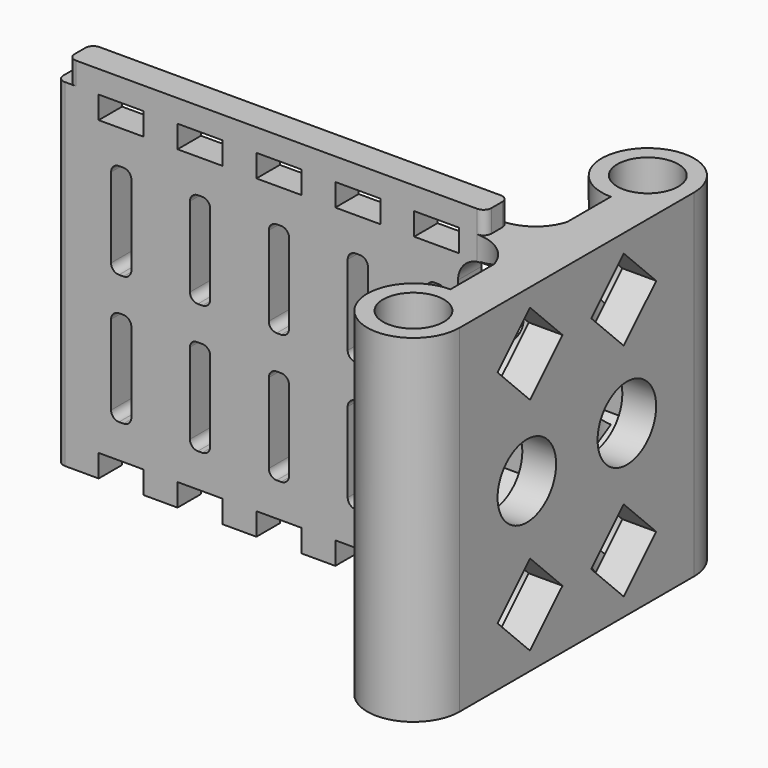
from build123d import *

# Parameters (mm, degrees)
F0_R     = 2.7
F1_DEPTH = 30
F3_DEPTH = 2
F4_R     = 3.25
F5_DEPTH = 25
F6_START = -3
F4_R_2   = 5
F6_DEPTH = 4.5
F7_W     = 4
F7_H     = 2
F8_DEPTH = 5


# Not quite as in the source:
# - a feature names something its author has since deleted; it is built from what else it names


with BuildPart() as f1:
    # F0 (on Top) → F1 (new body)
    with BuildSketch(Plane.XY):
        with BuildLine():
            ThreePointArc((14.1813559458, 17.5603501923), (17.0804937486, 18.7612123895), (18.2813559458, 21.6603501923))
            ThreePointArc((18.2813559458, 21.6603501923), (11.2822181429, 24.5594879952), (14.1813559458, 17.5603501923))
        make_face()
        with Locations((14.1813559458, 21.6603501923)):
            Circle(F0_R, mode=Mode.SUBTRACT)
        with BuildLine():
            Line((18.2813559458, -4.3396498077), (18.2813559458, 21.6603501923))
            ThreePointArc((18.2813559458, 21.6603501923), (17.0804937486, 18.7612123895), (14.1813559458, 17.5603501923))
            Line((14.1813559458, 17.5603501923), (14.1813559458, 12.7042196833))
            Line((14.1813559458, 12.7042196833), (14.1813559458, 4.6164807014))
            Line((14.1813559458, 4.6164807014), (14.1813559458, -0.2396498077))
            ThreePointArc((14.1813559458, -0.2396498077), (17.0804937486, -1.4405120048), (18.2813559458, -4.3396498077))
        make_face()
        with BuildLine():
            ThreePointArc((14.1813559458, -0.2396498077), (11.2822181429, -7.2387876105), (18.2813559458, -4.3396498077))
            ThreePointArc((18.2813559458, -4.3396498077), (17.0804937486, -1.4405120048), (14.1813559458, -0.2396498077))
        make_face()
        with Locations((14.1813559458, -4.3396498077)):
            Circle(F0_R, mode=Mode.SUBTRACT)
        with BuildLine():
            Line((14.1813559458, 4.6164807014), (14.1813559458, 12.7042196833))
            ThreePointArc((14.1813559458, 12.7042196833), (12.7845504547, 10.7211699819), (10.4813559458, 9.9603501923))
            ThreePointArc((10.4813559458, 9.9603501923), (10.9763306926, 9.7553249392), (11.1813559458, 9.2603501923))
            Line((11.1813559458, 9.2603501923), (11.1813559458, 8.0603501923))
            ThreePointArc((11.1813559458, 8.0603501923), (10.9763306926, 7.5653754455), (10.4813559458, 7.3603501923))
            ThreePointArc((10.4813559458, 7.3603501923), (12.7845504547, 6.5995304028), (14.1813559458, 4.6164807014))
        make_face()
        with BuildLine():
            ThreePointArc((11.1813559458, 9.2603501923), (10.9763306926, 9.7553249392), (10.4813559458, 9.9603501923))
            Line((10.4813559458, 9.9603501923), (-25.1186440542, 9.9603501923))
            ThreePointArc((-25.1186440542, 9.9603501923), (-25.6136188011, 9.7553249392), (-25.8186440542, 9.2603501923))
            Line((-25.8186440542, 9.2603501923), (-25.8186440542, 8.0603501923))
            ThreePointArc((-25.8186440542, 8.0603501923), (-25.6136188011, 7.5653754455), (-25.1186440542, 7.3603501923))
            Line((-25.1186440542, 7.3603501923), (10.4813559458, 7.3603501923))
            ThreePointArc((10.4813559458, 7.3603501923), (10.9763306926, 7.5653754455), (11.1813559458, 8.0603501923))
            Line((11.1813559458, 8.0603501923), (11.1813559458, 9.2603501923))
        make_face()
        with BuildLine():
            ThreePointArc((-25.8186440542, 9.2603501923), (-25.6136188011, 9.7553249392), (-25.1186440542, 9.9603501923))
            Line((-25.1186440542, 9.9603501923), (-26.1186440542, 9.9603501923))
            ThreePointArc((-26.1186440542, 9.9603501923), (-26.6136188011, 9.7553249392), (-26.8186440542, 9.2603501923))
            Line((-26.8186440542, 9.2603501923), (-26.8186440542, 8.0603501923))
            ThreePointArc((-26.8186440542, 8.0603501923), (-26.6136188011, 7.5653754455), (-26.1186440542, 7.3603501923))
            Line((-26.1186440542, 7.3603501923), (-25.1186440542, 7.3603501923))
            ThreePointArc((-25.1186440542, 7.3603501923), (-25.6136188011, 7.5653754455), (-25.8186440542, 8.0603501923))
            Line((-25.8186440542, 8.0603501923), (-25.8186440542, 9.2603501923))
        make_face()
    extrude(amount=F1_DEPTH)

    # F2 (on face) → F3 (join)
    with BuildSketch(Plane.XY.offset(30)):
        with BuildLine():
            Line((11.1813559458, 8.0603501923), (11.1813559458, 9.2603501923))
            ThreePointArc((11.1813559458, 9.2603501923), (10.9763306926, 9.7553249392), (10.4813559458, 9.9603501923))
            Line((10.4813559458, 9.9603501923), (-25.1186440542, 9.9603501923))
            ThreePointArc((-25.1186440542, 9.9603501923), (-25.6136188011, 9.7553249392), (-25.8186440542, 9.2603501923))
            Line((-25.8186440542, 9.2603501923), (-25.8186440542, 8.0603501923))
            ThreePointArc((-25.8186440542, 8.0603501923), (-25.6136188011, 7.5653754455), (-25.1186440542, 7.3603501923))
            Line((-25.1186440542, 7.3603501923), (10.4813559458, 7.3603501923))
            ThreePointArc((10.4813559458, 7.3603501923), (10.9763306926, 7.5653754455), (11.1813559458, 8.0603501923))
        make_face()
    extrude(amount=F3_DEPTH)

    # F4 (on face) → F5 (cut)
    with BuildSketch(Plane.YZ.offset(18.2813559458)):
        with Locations((14.2083470508, 15.0020234637)):
            Circle(F4_R)
        Polygon((7.0665947764, 24.8), (3.4603501923, 28.4062445841), (-0.1458943917, 24.8), (3.4603501923, 21.1937554159), align=None)
        Polygon((13.8603501923, 21.1937554159), (17.4665947764, 24.8), (13.8603501923, 28.4062445841), (10.2541056083, 24.8), align=None)
        with Locations((3.1123533338, 15.0020234637)):
            Circle(F4_R)
        Polygon((3.4603501923, 8.8062445841), (-0.1458943917, 5.2), (3.4603501923, 1.5937554159), (7.0665947764, 5.2), align=None)
        Polygon((13.8603501923, 1.5937554159), (17.4665947764, 5.2), (13.8603501923, 8.8062445841), (10.2541056083, 5.2), align=None)
    extrude(amount=-F5_DEPTH, mode=Mode.SUBTRACT)

    # F4 (on face) → F6 (cut)
    with BuildSketch(Plane.YZ.offset(18.2813559458).offset(F6_START)):
        Polygon((10.1083470508, 17.3691595674), (10.1083470508, 12.63488736), (14.2083470508, 10.2677512564), (18.3083470508, 12.63488736), (18.3083470508, 17.3691595674), (14.2083470508, 19.7362956711), align=None)
        with Locations((14.2083470508, 15.0020234637)):
            Circle(F4_R, mode=Mode.SUBTRACT)
        with Locations((3.4603501923, 24.8)):
            Circle(F4_R_2)
        Polygon((-0.1458943917, 24.8), (3.4603501923, 28.4062445841), (7.0665947764, 24.8), (3.4603501923, 21.1937554159), align=None, mode=Mode.SUBTRACT)
        with Locations((13.8603501923, 24.8)):
            Circle(F4_R_2)
        Polygon((13.8603501923, 28.4062445841), (17.4665947764, 24.8), (13.8603501923, 21.1937554159), (10.2541056083, 24.8), align=None, mode=Mode.SUBTRACT)
        Polygon((-0.9876466662, 12.63488736), (3.1123533338, 10.2677512564), (7.2123533338, 12.63488736), (7.2123533338, 17.3691595674), (3.1123533338, 19.7362956711), (-0.9876466662, 17.3691595674), align=None)
        with Locations((3.1123533338, 15.0020234637)):
            Circle(F4_R, mode=Mode.SUBTRACT)
        with Locations((3.4603501923, 5.2)):
            Circle(F4_R_2)
        Polygon((3.4603501923, 1.5937554159), (-0.1458943917, 5.2), (3.4603501923, 8.8062445841), (7.0665947764, 5.2), align=None, mode=Mode.SUBTRACT)
        with Locations((13.8603501923, 5.2)):
            Circle(F4_R_2)
        Polygon((13.8603501923, 8.8062445841), (17.4665947764, 5.2), (13.8603501923, 1.5937554159), (10.2541056083, 5.2), align=None, mode=Mode.SUBTRACT)
    extrude(amount=-F6_DEPTH, mode=Mode.SUBTRACT)

    # F7 (on face) → F8 (cut, symmetric)
    with BuildSketch(Plane.XZ.offset(-7.3603501923)):
        with Locations((-21.1186440542, 29)):
            Rectangle(F7_W, F7_H)
        with Locations((-14.1186440542, 29)):
            Rectangle(F7_W, F7_H)
        with Locations((-7.1186440542, 29)):
            Rectangle(F7_W, F7_H)
        with Locations((-0.1186440542, 29)):
            Rectangle(F7_W, F7_H)
        with Locations((6.8813559458, 29)):
            Rectangle(F7_W, F7_H)
        with BuildLine():
            ThreePointArc((7.7813559458, 24.3), (7.5763306926, 24.7949747468), (7.0813559458, 25))
            Line((7.0813559458, 25), (6.6813559458, 25))
            ThreePointArc((6.6813559458, 25), (6.1863811989, 24.7949747468), (5.9813559458, 24.3))
            Line((5.9813559458, 24.3), (5.9813559458, 17.2))
            ThreePointArc((5.9813559458, 17.2), (6.1863811989, 16.7050252532), (6.6813559458, 16.5))
            Line((6.6813559458, 16.5), (7.0813559458, 16.5))
            ThreePointArc((7.0813559458, 16.5), (7.5763306926, 16.7050252532), (7.7813559458, 17.2))
            Line((7.7813559458, 17.2), (7.7813559458, 24.3))
        make_face()
        with BuildLine():
            Line((0.0813559458, 25), (-0.3186440542, 25))
            ThreePointArc((-0.3186440542, 25), (-0.8136188011, 24.7949747468), (-1.0186440542, 24.3))
            Line((-1.0186440542, 24.3), (-1.0186440542, 17.2))
            ThreePointArc((-1.0186440542, 17.2), (-0.8136188011, 16.7050252532), (-0.3186440542, 16.5))
            Line((-0.3186440542, 16.5), (0.0813559458, 16.5))
            ThreePointArc((0.0813559458, 16.5), (0.5763306926, 16.7050252532), (0.7813559458, 17.2))
            Line((0.7813559458, 17.2), (0.7813559458, 24.3))
            ThreePointArc((0.7813559458, 24.3), (0.5763306926, 24.7949747468), (0.0813559458, 25))
        make_face()
        with BuildLine():
            ThreePointArc((-6.2186440542, 24.3), (-6.4236693074, 24.7949747468), (-6.9186440542, 25))
            Line((-6.9186440542, 25), (-7.3186440542, 25))
            ThreePointArc((-7.3186440542, 25), (-7.8136188011, 24.7949747468), (-8.0186440542, 24.3))
            Line((-8.0186440542, 24.3), (-8.0186440542, 17.2))
            ThreePointArc((-8.0186440542, 17.2), (-7.8136188011, 16.7050252532), (-7.3186440542, 16.5))
            Line((-7.3186440542, 16.5), (-6.9186440542, 16.5))
            ThreePointArc((-6.9186440542, 16.5), (-6.4236693074, 16.7050252532), (-6.2186440542, 17.2))
            Line((-6.2186440542, 17.2), (-6.2186440542, 24.3))
        make_face()
        with BuildLine():
            ThreePointArc((-13.2186440542, 24.3), (-13.4236693074, 24.7949747468), (-13.9186440542, 25))
            Line((-13.9186440542, 25), (-14.3186440542, 25))
            ThreePointArc((-14.3186440542, 25), (-14.8136188011, 24.7949747468), (-15.0186440542, 24.3))
            Line((-15.0186440542, 24.3), (-15.0186440542, 17.2))
            ThreePointArc((-15.0186440542, 17.2), (-14.8136188011, 16.7050252532), (-14.3186440542, 16.5))
            Line((-14.3186440542, 16.5), (-13.9186440542, 16.5))
            ThreePointArc((-13.9186440542, 16.5), (-13.4236693074, 16.7050252532), (-13.2186440542, 17.2))
            Line((-13.2186440542, 17.2), (-13.2186440542, 24.3))
        make_face()
        with BuildLine():
            ThreePointArc((-20.2186440542, 24.3), (-20.4236693074, 24.7949747468), (-20.9186440542, 25))
            Line((-20.9186440542, 25), (-21.3186440542, 25))
            ThreePointArc((-21.3186440542, 25), (-21.8136188011, 24.7949747468), (-22.0186440542, 24.3))
            Line((-22.0186440542, 24.3), (-22.0186440542, 17.2))
            ThreePointArc((-22.0186440542, 17.2), (-21.8136188011, 16.7050252532), (-21.3186440542, 16.5))
            Line((-21.3186440542, 16.5), (-20.9186440542, 16.5))
            ThreePointArc((-20.9186440542, 16.5), (-20.4236693074, 16.7050252532), (-20.2186440542, 17.2))
            Line((-20.2186440542, 17.2), (-20.2186440542, 24.3))
        make_face()
        with Locations((-14.1186440542, 1)):
            Rectangle(F7_W, F7_H)
        with Locations((-7.1186440542, 1)):
            Rectangle(F7_W, F7_H)
        with Locations((-0.1186440542, 1)):
            Rectangle(F7_W, F7_H)
        with Locations((6.8813559458, 1)):
            Rectangle(F7_W, F7_H)
        with Locations((-21.1186440542, 1)):
            Rectangle(F7_W, F7_H)
        with BuildLine():
            Line((10.4813559458, 21.7720537787), (10.4813559458, 27.8578661878))
            ThreePointArc((10.4813559458, 27.8578661878), (9.264780857, 27.1843346755), (8.7813559458, 25.8804941945))
            Line((8.7813559458, 25.8804941945), (8.7813559458, 23.7494257721))
            ThreePointArc((8.7813559458, 23.7494257721), (9.264780857, 22.445585291), (10.4813559458, 21.7720537787))
        make_face()
        with BuildLine():
            ThreePointArc((10.7813559458, 27.8804941945), (10.630929862, 27.8748291697), (10.4813559458, 27.8578661878))
            Line((10.4813559458, 27.8578661878), (10.4813559458, 21.7720537787))
            ThreePointArc((10.4813559458, 21.7720537787), (10.630929862, 21.7550907969), (10.7813559458, 21.7494257721))
            Line((10.7813559458, 21.7494257721), (11.7813559458, 21.7494257721))
            ThreePointArc((11.7813559458, 21.7494257721), (13.1955695081, 22.3352122097), (13.7813559458, 23.7494257721))
            Line((13.7813559458, 23.7494257721), (13.7813559458, 25.8804941945))
            ThreePointArc((13.7813559458, 25.8804941945), (13.1955695081, 27.2947077568), (11.7813559458, 27.8804941945))
            Line((11.7813559458, 27.8804941945), (10.7813559458, 27.8804941945))
        make_face()
        with BuildLine():
            Line((-21.3186440542, 5), (-20.9186440542, 5))
            ThreePointArc((-20.9186440542, 5), (-20.4236693074, 5.2050252532), (-20.2186440542, 5.7))
            Line((-20.2186440542, 5.7), (-20.2186440542, 12.8))
            ThreePointArc((-20.2186440542, 12.8), (-20.4236693074, 13.2949747468), (-20.9186440542, 13.5))
            Line((-20.9186440542, 13.5), (-21.3186440542, 13.5))
            ThreePointArc((-21.3186440542, 13.5), (-21.8136188011, 13.2949747468), (-22.0186440542, 12.8))
            Line((-22.0186440542, 12.8), (-22.0186440542, 5.7))
            ThreePointArc((-22.0186440542, 5.7), (-21.8136188011, 5.2050252532), (-21.3186440542, 5))
        make_face()
        with BuildLine():
            Line((-14.3186440542, 5), (-13.9186440542, 5))
            ThreePointArc((-13.9186440542, 5), (-13.4236693074, 5.2050252532), (-13.2186440542, 5.7))
            Line((-13.2186440542, 5.7), (-13.2186440542, 12.8))
            ThreePointArc((-13.2186440542, 12.8), (-13.4236693074, 13.2949747468), (-13.9186440542, 13.5))
            Line((-13.9186440542, 13.5), (-14.4186440542, 13.5))
            ThreePointArc((-14.4186440542, 13.5), (-14.8429081229, 13.3242640687), (-15.0186440542, 12.9))
            Line((-15.0186440542, 12.9), (-15.0186440542, 5.7))
            ThreePointArc((-15.0186440542, 5.7), (-14.8136188011, 5.2050252532), (-14.3186440542, 5))
        make_face()
        with BuildLine():
            Line((-7.3186440542, 5), (-6.9186440542, 5))
            ThreePointArc((-6.9186440542, 5), (-6.4236693074, 5.2050252532), (-6.2186440542, 5.7))
            Line((-6.2186440542, 5.7), (-6.2186440542, 12.8))
            ThreePointArc((-6.2186440542, 12.8), (-6.4236693074, 13.2949747468), (-6.9186440542, 13.5))
            Line((-6.9186440542, 13.5), (-7.3186440542, 13.5))
            ThreePointArc((-7.3186440542, 13.5), (-7.8136188011, 13.2949747468), (-8.0186440542, 12.8))
            Line((-8.0186440542, 12.8), (-8.0186440542, 5.7))
            ThreePointArc((-8.0186440542, 5.7), (-7.8136188011, 5.2050252532), (-7.3186440542, 5))
        make_face()
        with BuildLine():
            ThreePointArc((-1.0186440542, 5.7), (-0.8136188011, 5.2050252532), (-0.3186440542, 5))
            Line((-0.3186440542, 5), (0.0813559458, 5))
            ThreePointArc((0.0813559458, 5), (0.5763306926, 5.2050252532), (0.7813559458, 5.7))
            Line((0.7813559458, 5.7), (0.7813559458, 12.8))
            ThreePointArc((0.7813559458, 12.8), (0.5763306926, 13.2949747468), (0.0813559458, 13.5))
            Line((0.0813559458, 13.5), (-0.3186440542, 13.5))
            ThreePointArc((-0.3186440542, 13.5), (-0.8136188011, 13.2949747468), (-1.0186440542, 12.8))
            Line((-1.0186440542, 12.8), (-1.0186440542, 5.7))
        make_face()
        with BuildLine():
            Line((6.6813559458, 5), (7.0813559458, 5))
            ThreePointArc((7.0813559458, 5), (7.5763306926, 5.2050252532), (7.7813559458, 5.7))
            Line((7.7813559458, 5.7), (7.7813559458, 12.8))
            ThreePointArc((7.7813559458, 12.8), (7.5763306926, 13.2949747468), (7.0813559458, 13.5))
            Line((7.0813559458, 13.5), (6.6813559458, 13.5))
            ThreePointArc((6.6813559458, 13.5), (6.1863811989, 13.2949747468), (5.9813559458, 12.8))
            Line((5.9813559458, 12.8), (5.9813559458, 5.7))
            ThreePointArc((5.9813559458, 5.7), (6.1863811989, 5.2050252532), (6.6813559458, 5))
        make_face()
    extrude(amount=F8_DEPTH, both=True, mode=Mode.SUBTRACT)


solid = f1.part
